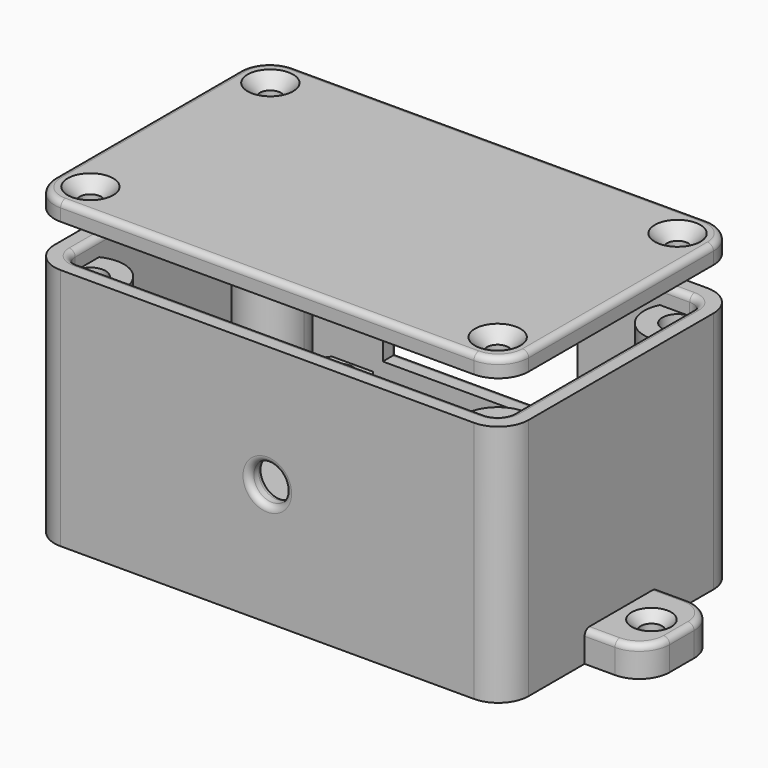
from build123d import *

# Parameters (mm, degrees)
F0_W      = 72
F0_H      = 42
F1_DEPTH  = 40
F2_DEPTH  = 3
F3_R      = 2.5
F3_R_2    = 4.5
F4_DEPTH  = 9
F5_W      = 32
F5_H      = 17
F6_DEPTH  = 25
F7_DEPTH  = 34
F8_R      = 5
F9_R      = 2.49999
F10_R     = 1
F0_W_2    = 10
F0_H_2    = 15
F0_R      = 1.75
F11_DEPTH = 5
F12_R     = 5
F13_R     = 1
F14_SIZE  = 1.5
F16_W     = 78
F16_H     = 48
F16_W_2   = 72
F16_H_2   = 42
F17_DEPTH = 3
F16_R     = 1.75
F18_DEPTH = 5
F19_SIZE  = 2
F20_R     = 5
F21_R     = 2.5
F22_R     = 1
F23_R     = 3
F24_DEPTH = 25
F25_R     = 1
F26_R     = 1
F27_R     = 1


# Not quite as in the source:
# - a fillet or chamfer is up to 0.001 mm smaller than in the source, because OpenCascade refuses the exact size


with BuildPart() as f1:
    # F0 (on Top) → F1 (new body)
    with BuildSketch(Plane.XY):
        Polygon((39, 24), (-39, 24), (-39, 7.5), (-39, -7.5), (-39, -24), (39, -24), (39, -7.5), (39, 7.5), align=None)
        Rectangle(F0_W, F0_H, mode=Mode.SUBTRACT)
    extrude(amount=F1_DEPTH)

    # F0 (on Top) → F2 (join)
    with BuildSketch(Plane.XY):
        Rectangle(F0_W, F0_H)
    extrude(amount=F2_DEPTH)

    # F3 (on face) → F4 (join)
    with BuildSketch(Plane.XY.offset(3)):
        with BuildLine():
            ThreePointArc((-25.3541019662, 21), (-23.605699404, 13.7962243847), (-17.5, 18))
            ThreePointArc((-17.5, 18), (-17.7962243847, 19.605699404), (-18.6458980338, 21))
            Line((-18.6458980338, 21), (-25.3541019662, 21))
        make_face()
        with Locations((-22, 18)):
            Circle(F3_R, mode=Mode.SUBTRACT)
        with Locations((-22, -13)):
            Circle(F3_R_2)
        with Locations((-22, -13)):
            Circle(F3_R, mode=Mode.SUBTRACT)
        with Locations((21, -13)):
            Circle(F3_R_2)
        with Locations((21, -13)):
            Circle(F3_R, mode=Mode.SUBTRACT)
        with BuildLine():
            Line((24.3541019662, 21), (17.6458980338, 21))
            ThreePointArc((17.6458980338, 21), (19.394300596, 13.7962243847), (25.5, 18))
            ThreePointArc((25.5, 18), (25.2037756153, 19.605699404), (24.3541019662, 21))
        make_face()
        with Locations((21, 18)):
            Circle(F3_R, mode=Mode.SUBTRACT)
    extrude(amount=F4_DEPTH)

    # F5 (on face) → F6 (cut)
    with BuildSketch(Plane.XZ.offset(-21)):
        with Locations((-1, 22.5)):
            Rectangle(F5_W, F5_H)
    extrude(amount=-F6_DEPTH, mode=Mode.SUBTRACT)

    # F3 (on face) → F7 (join)
    with BuildSketch(Plane.XY.offset(3)):
        with BuildLine():
            ThreePointArc((-28, -18.5), (-30.6277186767, -13.8095842402), (-36, -13.6010205144))
            Line((-36, -13.6010205144), (-36, -18.5))
            ThreePointArc((-36, -18.5), (-33.5, -16), (-31, -18.5))
            ThreePointArc((-31, -18.5), (-31.732233047, -20.267766953), (-33.5, -21))
            Line((-33.5, -21), (-28.6010205144, -21))
            ThreePointArc((-28.6010205144, -21), (-28.1523656085, -19.7856151892), (-28, -18.5))
        make_face()
        with BuildLine():
            Line((36, -18.5), (36, -13.6010205144))
            ThreePointArc((36, -13.6010205144), (29.6109127035, -14.6109127035), (28.6010205144, -21))
            Line((28.6010205144, -21), (33.5000000781, -21))
            ThreePointArc((33.5000000781, -21), (31.7322330194, -16.7322330746), (36, -18.5))
        make_face()
        with BuildLine():
            Line((33.5, 21), (28.6010205144, 21))
            ThreePointArc((28.6010205144, 21), (29.6109127035, 14.6109127035), (36, 13.6010205144))
            Line((36, 13.6010205144), (36, 18.5))
            ThreePointArc((36, 18.5), (31.732233047, 16.732233047), (33.5, 21))
        make_face()
        with BuildLine():
            ThreePointArc((-28, 18.5), (-28.1523656085, 19.7856151892), (-28.6010205144, 21))
            Line((-28.6010205144, 21), (-33.5000000781, 21))
            ThreePointArc((-33.5000000781, 21), (-31.7322330746, 20.2677669806), (-31, 18.5))
            ThreePointArc((-31, 18.5), (-33.5, 16), (-36, 18.5))
            Line((-36, 18.5), (-36, 13.6010205144))
            ThreePointArc((-36, 13.6010205144), (-30.6277186767, 13.8095842402), (-28, 18.5))
        make_face()
    extrude(amount=F7_DEPTH)

    # F8
    f8_edges = [f1.edges().sort_by_distance(p)[0] for p in [
        (-39, -24, 20),
        (39, -24, 20),
        (39, 24, 20),
        (-39, 24, 20),
    ]]
    fillet(f8_edges, radius=F8_R)

    # F9 (radius 2.5 in the source; OpenCascade refuses exactly that, so slightly less here)
    f9_edges = [f1.edges().sort_by_distance(p)[0] for p in [
        (-36, -21, 21.5),
        (-36, 21, 21.5),
        (36, -21, 21.5),
        (36, 21, 21.5),
    ]]
    fillet(f9_edges, radius=F9_R)

    # F10
    f10_edges = [f1.edges().sort_by_distance(p)[0] for p in [
        (-1, 24, 31),
        (-17, 24, 22.5),
        (-1, 24, 14),
        (15, 24, 22.5),
    ]]
    fillet(f10_edges, radius=F10_R)

    # F0 (on Top) → F11 (join)
    with BuildSketch(Plane.XY):
        with Locations((44, 0)):
            Rectangle(F0_W_2, F0_H_2)
        with Locations((44, 0)):
            Circle(F0_R, mode=Mode.SUBTRACT)
        with Locations((-44, 0)):
            Rectangle(F0_W_2, F0_H_2)
        with Locations((-44, 0)):
            Circle(F0_R, mode=Mode.SUBTRACT)
    extrude(amount=F11_DEPTH)

    # F12
    f12_edges = [f1.edges().sort_by_distance(p)[0] for p in [
        (49, 7.5, 2.5),
        (-49, 7.5, 2.5),
        (-49, -7.5, 2.5),
        (49, -7.5, 2.5),
    ]]
    fillet(f12_edges, radius=F12_R)

    # F13
    f13_edges = [f1.edges().sort_by_distance(p)[0] for p in [
        (-41.5, 7.5, 5),
        (41.5, -7.5, 5),
    ]]
    fillet(f13_edges, radius=F13_R)

    # F14
    f14_edges = [f1.edges().sort_by_distance(p)[0] for p in [
        (42.25, 0, 5),
        (-45.75, 0, 5),
    ]]
    chamfer(f14_edges, length=F14_SIZE)

    # F23 (on face) → F24 (cut)
    with BuildSketch(Plane.XZ.offset(24)):
        with Locations((0, 20)):
            Circle(F23_R)
    extrude(amount=-F24_DEPTH, mode=Mode.SUBTRACT)

    # F25
    f25_edges = [f1.edges().sort_by_distance(p)[0] for p in [
        (-3, -24, 20),
        (-3, -21, 20),
    ]]
    fillet(f25_edges, radius=F25_R)

    # F27
    f27_edges = [f1.edges().sort_by_distance(p)[0] for p in [
        (0, 21, 40),
    ]]
    fillet(f27_edges, radius=F27_R)


with BuildPart() as f17:
    # F16 (on offset) → F17 (new body)
    with BuildSketch(Plane.XY.offset(50)):
        Rectangle(F16_W, F16_H)
        Rectangle(F16_W_2, F16_H_2, mode=Mode.SUBTRACT)
    extrude(amount=-F17_DEPTH)

    # F16 (on offset) → F18 (join)
    with BuildSketch(Plane.XY.offset(50)):
        Rectangle(F16_W_2, F16_H_2)
        with Locations((-33.5, -18.5)):
            Circle(F16_R, mode=Mode.SUBTRACT)
        with Locations((33.5, -18.5)):
            Circle(F16_R, mode=Mode.SUBTRACT)
        with Locations((-33.5, 18.5)):
            Circle(F16_R, mode=Mode.SUBTRACT)
        with Locations((33.5, 18.5)):
            Circle(F16_R, mode=Mode.SUBTRACT)
    extrude(amount=-F18_DEPTH)

    # F19
    f19_edges = [f17.edges().sort_by_distance(p)[0] for p in [
        (-35.25, 18.5, 50),
        (-35.25, -18.5, 50),
        (31.75, 18.5, 50),
        (31.75, -18.5, 50),
    ]]
    chamfer(f19_edges, length=F19_SIZE)

    # F20
    f20_edges = [f17.edges().sort_by_distance(p)[0] for p in [
        (-39, -24, 48.5),
        (-39, 24, 48.5),
        (39, 24, 48.5),
        (39, -24, 48.5),
    ]]
    fillet(f20_edges, radius=F20_R)

    # F21
    f21_edges = [f17.edges().sort_by_distance(p)[0] for p in [
        (36, -21, 46),
        (36, 21, 46),
        (-36, 21, 46),
        (-36, -21, 46),
    ]]
    fillet(f21_edges, radius=F21_R)

    # F22
    f22_edges = [f17.edges().sort_by_distance(p)[0] for p in [
        (39, 0, 50),
    ]]
    fillet(f22_edges, radius=F22_R)

    # F26
    f26_edges = [f17.edges().sort_by_distance(p)[0] for p in [
        (0, 21, 45),
    ]]
    fillet(f26_edges, radius=F26_R)


solid = Compound([f1.part, f17.part])
